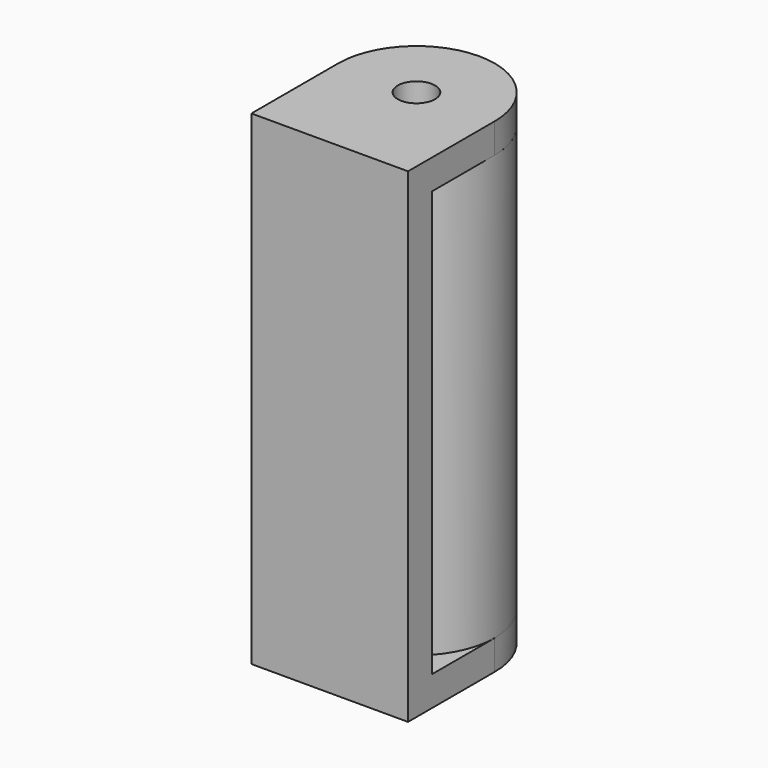
from build123d import *

# Parameters (mm, degrees)
F0_R     = 5.25
F1_DEPTH = 14.25
F3_DEPTH = 2
F4_W     = 10.5
F4_H     = 2
F5_DEPTH = 16.25
F6_R     = 1.25
F7_DEPTH = 2


with BuildPart() as f1:
    # F0 (on Top) → F1 (new body, symmetric)
    with BuildSketch(Plane.XY):
        Circle(F0_R)
    extrude(amount=F1_DEPTH, both=True)


with BuildPart() as f3:
    # F2 (on face) → F3 (new body)
    with BuildSketch(Plane.XY.offset(14.25)):
        with BuildLine():
            Line((5.25, -5.2667460404), (5.25, 0))
            ThreePointArc((5.25, 0), (0, 5.25), (-5.25, 0))
            Line((-5.25, 0), (-5.25, -5.2667460404))
            Line((-5.25, -5.2667460404), (5.25, -5.2667460404))
        make_face()
    extrude(amount=F3_DEPTH)

    # F4 (on face) → F5 (join, through all)
    with BuildSketch(Plane.XY.offset(16.25)):
        with Locations((0, -6.2667460404)):
            Rectangle(F4_W, F4_H)
    extrude(amount=-F5_DEPTH)

    # F6 (on face) → F7 (cut, through all)
    with BuildSketch(Plane.XY.offset(16.25)):
        Circle(F6_R)
    extrude(amount=-F7_DEPTH, mode=Mode.SUBTRACT)

    # F8: F3 across plane


with BuildPart() as f3_1:
    add(f3.part)
    add(f3.part.mirror(Plane.XY))


solid = Compound([f1.part, f3_1.part])
